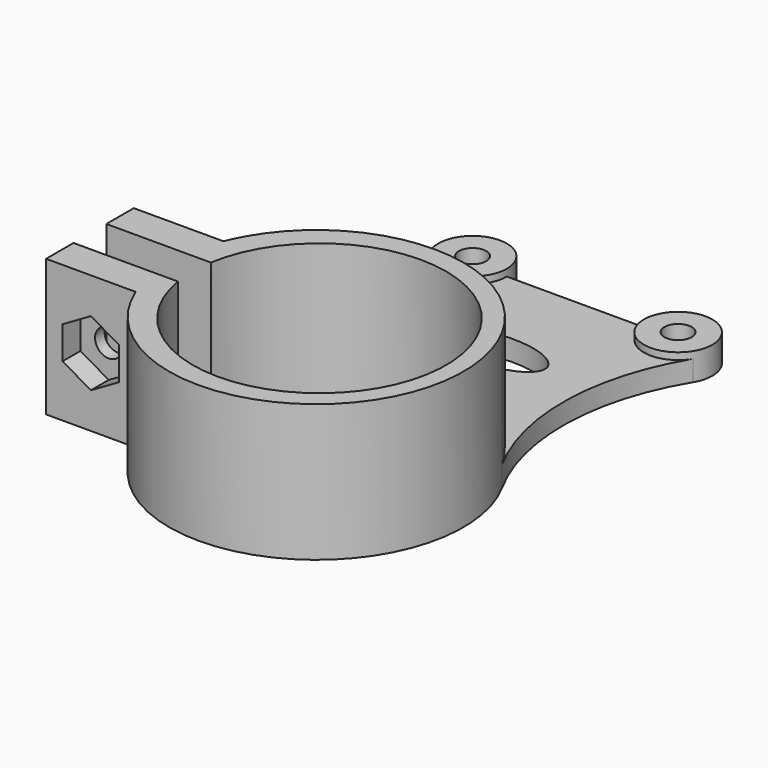
from build123d import *

# Parameters (mm, degrees)
F1_DEPTH = 20
F0_R     = 2
F2_DEPTH = 3
F3_DEPTH = 4
F5_DEPTH = 3.25
F6_R     = 2
F7_DEPTH = 29.5010001


# Not quite as in the source:
# - a feature names something its author has since deleted; it is built from what else it names


with BuildPart() as f1:
    # F0 (on Top) → F1 (new body)
    with BuildSketch(Plane.XY):
        with BuildLine():
            ThreePointArc((-18.2551362635, 3.1646558729), (18.5, 0.1646558729), (-18.2551362635, -2.8353441271))
            Line((-18.2551362635, -2.8353441271), (-21.289668856, -2.8353441271))
            Line((-21.289668856, -2.8353441271), (-33.5, -2.8353441271))
            Line((-33.5, -2.8353441271), (-33.5, -5.8353441271))
            Line((-33.5, -5.8353441271), (-33.5, -7.8353441271))
            Line((-33.5, -7.8353441271), (-20.4217309456, -7.8353441271))
            ThreePointArc((-20.4217309456, -7.8353441271), (8.7176252261, -19.2755005117), (18.3885107603, 10.4978639134))
            ThreePointArc((18.3885107603, 10.4978639134), (-0.3478610365, 21.6643338769), (-19.2053350681, 10.7036152553))
            ThreePointArc((-19.2053350681, 10.7036152553), (-19.8551354356, 9.4540669672), (-20.4217309456, 8.1646558729))
            Line((-20.4217309456, 8.1646558729), (-33.5, 8.1646558729))
            Line((-33.5, 8.1646558729), (-33.5, 6.1646558729))
            Line((-33.5, 6.1646558729), (-33.5, 3.1646558729))
            Line((-33.5, 3.1646558729), (-21.289668856, 3.1646558729))
            Line((-21.289668856, 3.1646558729), (-18.2551362635, 3.1646558729))
        make_face()
    extrude(amount=F1_DEPTH)

    # F0 (on Top) → F2 (join)
    with BuildSketch(Plane.XY):
        with BuildLine():
            ThreePointArc((-19.2053350681, 10.7036152553), (-0.3478610365, 21.6643338769), (18.3885107603, 10.4978639134))
            ThreePointArc((18.3885107603, 10.4978639134), (14.2120337074, 27.5685018888), (19.1172770705, 44.4441716239))
            ThreePointArc((19.1172770705, 44.4441716239), (13.4958098431, 42.2172179553), (9.8397882001, 47.0332040616))
            Line((9.8397882001, 47.0332040616), (-10.1602117999, 47.0332040616))
            ThreePointArc((-10.1602117999, 47.0332040616), (-13.8544265436, 42.2067224379), (-19.4781817457, 44.512264644))
            ThreePointArc((-19.4781817457, 44.512264644), (-14.8414845345, 27.6442586076), (-19.2053350681, 10.7036152553))
        make_face()
        with BuildLine():
            add(Edge.make_bspline(
                [(7.5, 31.9373905659), (7.5, 37.9995683924), (-3.75, 34.9684794791), (-15, 31.9373905659), (-3.75, 28.9063016526), (7.5, 25.8752127394), (7.5, 31.9373905659)],
                knots=[0, 0, 0, 2.0943951024, 2.0943951024, 4.1887902048, 4.1887902048, 6.2831853072, 6.2831853072, 6.2831853072], degree=2, weights=[1, 0.5, 1, 0.5, 1, 0.5, 1]))
        make_face(mode=Mode.SUBTRACT)
        with BuildLine():
            ThreePointArc((-10.1602117999, 47.0332040616), (-16.4659970562, 51.8596856854), (-19.4781817457, 44.512264644))
            ThreePointArc((-19.4781817457, 44.512264644), (-13.8544265436, 42.2067224379), (-10.1602117999, 47.0332040616))
        make_face()
        with Locations((-15.1602117999, 47.0332040616)):
            Circle(F0_R, mode=Mode.SUBTRACT)
        with BuildLine():
            ThreePointArc((9.8397882001, 47.0332040616), (13.4958098431, 42.2172179553), (19.1172770705, 44.4441716239))
            ThreePointArc((19.1172770705, 44.4441716239), (19.6557743064, 45.6892257046), (19.8397882001, 47.0332040616))
            ThreePointArc((19.8397882001, 47.0332040616), (14.8397882001, 52.0332040616), (9.8397882001, 47.0332040616))
        make_face()
        with BuildLine():
            ThreePointArc((16.8397882001, 47.0332040616), (14.8397882001, 45.0332040616), (12.8397882001, 47.0332040616))
            ThreePointArc((12.8397882001, 47.0332040616), (14.8397882001, 49.0332040616), (16.8397882001, 47.0332040616))
        make_face(mode=Mode.SUBTRACT)
    extrude(amount=F2_DEPTH)

    # F0 (on Top) → F3 (join)
    with BuildSketch(Plane.XY):
        with BuildLine():
            ThreePointArc((-10.1602117999, 47.0332040616), (-16.4659970562, 51.8596856854), (-19.4781817457, 44.512264644))
            ThreePointArc((-19.4781817457, 44.512264644), (-13.8544265436, 42.2067224379), (-10.1602117999, 47.0332040616))
        make_face()
        with Locations((-15.1602117999, 47.0332040616)):
            Circle(F0_R, mode=Mode.SUBTRACT)
        with BuildLine():
            ThreePointArc((9.8397882001, 47.0332040616), (13.4958098431, 42.2172179553), (19.1172770705, 44.4441716239))
            ThreePointArc((19.1172770705, 44.4441716239), (19.6557743064, 45.6892257046), (19.8397882001, 47.0332040616))
            ThreePointArc((19.8397882001, 47.0332040616), (14.8397882001, 52.0332040616), (9.8397882001, 47.0332040616))
        make_face()
        with BuildLine():
            ThreePointArc((16.8397882001, 47.0332040616), (14.8397882001, 45.0332040616), (12.8397882001, 47.0332040616))
            ThreePointArc((12.8397882001, 47.0332040616), (14.8397882001, 49.0332040616), (16.8397882001, 47.0332040616))
        make_face(mode=Mode.SUBTRACT)
    extrude(amount=F3_DEPTH)

    # F4 (on face) → F5 (cut)
    with BuildSketch(Plane.XZ.offset(7.8353441271)):
        Polygon((-31.0858654728, 12.3815698604), (-31.0858654728, 7.6184301396), (-26.9608654728, 5.2368602792), (-22.8358654728, 7.6184301396), (-22.8358654728, 12.3815698604), (-26.9608654728, 14.7631397208), align=None)
    extrude(amount=-F5_DEPTH, mode=Mode.SUBTRACT)

    # F6 (on face) → F7 (cut, through all)
    with BuildSketch(Plane(origin=(0, 8.1646558729, 0), x_dir=(-1, 0, 0), z_dir=(0, 1, 0))):
        with Locations((26.9608654728, 10)):
            Circle(F6_R)
    extrude(amount=-F7_DEPTH, mode=Mode.SUBTRACT)


solid = f1.part
